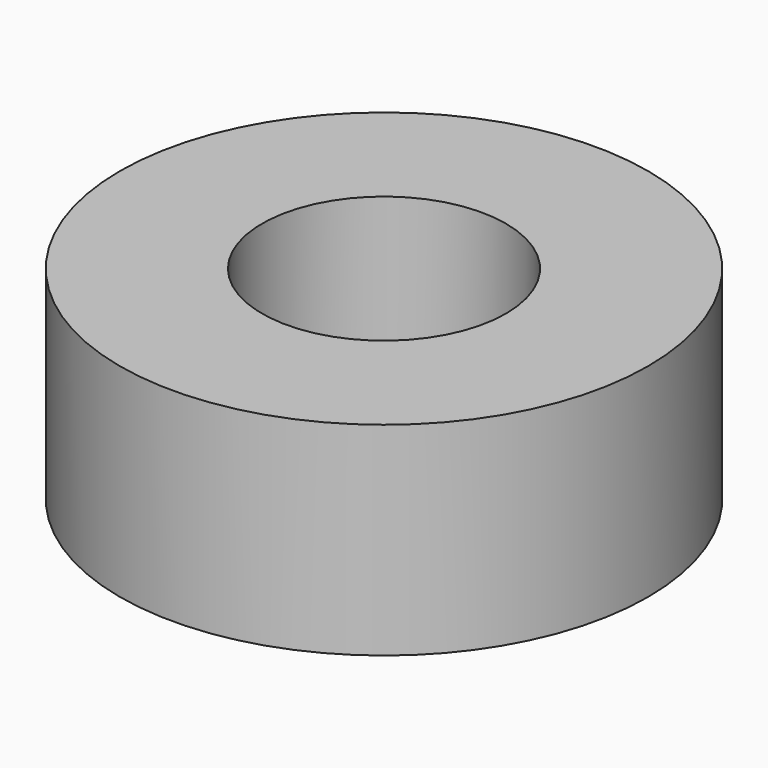
from build123d import *

# Parameters (mm, degrees)
F0_R     = 10.31875
F0_R_2   = 4.7625
F1_DEPTH = 7.9375


# Not quite as in the source:
# - a length typed as a fraction of an inch, garbled in the dataset ("3 / 203.2 mm" for 3/8 in), is restored


with BuildPart() as f1:
    # F0 (on Top) → F1 (new body)
    with BuildSketch(Plane.XY):
        Circle(F0_R)
        Circle(F0_R_2, mode=Mode.SUBTRACT)
    extrude(amount=F1_DEPTH)


solid = f1.part
